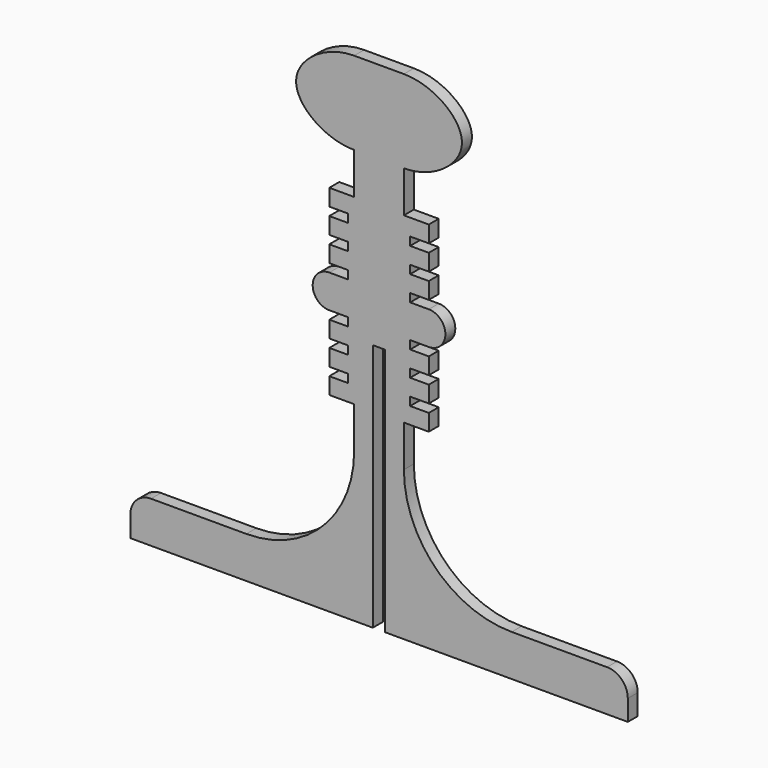
from build123d import *

# Parameters (mm, degrees)
F1_DEPTH = 3


# Not quite as in the source:
# - a feature names something its author has since deleted; it is built from what else it names


with BuildPart() as f1:
    # F0 (on Front) → F1 (new body)
    with BuildSketch(Plane.XZ):
        with BuildLine():
            Line((-1.5, 100), (-1.5, 120))
            Line((-1.5, 120), (-6, 120))
            add(Edge.make_bspline(
                [(-6, 120), (-13.1006129086, 120), (-20, 115.0061184168), (-20, 110)],
                knots=[0, 0, 0, 0, 0.5, 0.5, 0.5, 0.5], degree=3))
            add(Edge.make_bspline(
                [(-20, 110), (-20, 104.9938815832), (-13.1006129086, 99.9755263329), (-6, 100)],
                knots=[0.5, 0.5, 0.5, 0.5, 1, 1, 1, 1], degree=3))
            Line((-6, 100), (-1.5, 100))
        make_face()
        Polygon((-12, 68), (-6, 68), (-6, 90), (-12, 90), (-12, 86), (-7.5, 86), (-7.5, 84), (-12, 84), (-12, 80), (-7.5, 80), (-7.5, 78), (-12, 78), (-12, 74), (-7.5, 74), (-7.5, 72), (-12, 72), align=None)
        Polygon((-12, 46), (-6, 46), (-6, 68), (-12, 68), (-12, 64), (-7.5, 64), (-7.5, 62), (-12, 62), (-12, 58), (-7.5, 58), (-7.5, 56), (-12, 56), (-12, 52), (-7.5, 52), (-7.5, 50), (-12, 50), align=None)
        with BuildLine():
            Line((-12, 64), (-12, 68))
            Line((-12, 68), (-12, 72))
            ThreePointArc((-12, 72), (-16, 68), (-12, 64))
        make_face()
        with BuildLine():
            Line((12, 68), (12, 64))
            ThreePointArc((12, 64), (16, 68), (12, 72))
            Line((12, 72), (12, 68))
        make_face()
        Polygon((6, 90), (6, 46), (12, 46), (12, 50), (7.5, 50), (7.5, 52), (12, 52), (12, 56), (7.5, 56), (7.5, 58), (12, 58), (12, 62), (7.5, 62), (7.5, 64), (12, 64), (12, 68), (12, 72), (7.5, 72), (7.5, 74), (12, 74), (12, 78), (7.5, 78), (7.5, 80), (12, 80), (12, 84), (7.5, 84), (7.5, 86), (12, 86), (12, 90), align=None)
        with BuildLine():
            Line((1.5, 0), (60, 0))
            Line((60, 0), (60, 5))
            ThreePointArc((60, 5), (58.5355339059, 8.5355339059), (55, 10))
            Line((55, 10), (32, 10))
            ThreePointArc((32, 10), (13.6152236891, 17.6152236891), (6, 36))
            Line((6, 36), (6, 46))
            Line((6, 46), (6, 90))
            Line((6, 90), (6, 100))
            add(Edge.make_bspline(
                [(6, 120), (13.1006129086, 120), (26.8993870914, 110.0122368336), (13.1006129086, 99.9755263329), (6, 100)],
                knots=[0, 0, 0, 0, 0.5, 1, 1, 1, 1], degree=3))
            Line((6, 120), (1.5, 120))
            Line((1.5, 120), (-1.5, 120))
            Line((-1.5, 120), (-1.5, 100))
            Line((-1.5, 100), (-6, 100))
            Line((-6, 100), (-6, 90))
            Line((-6, 90), (-6, 68))
            Line((-6, 68), (-6, 46))
            Line((-6, 46), (-6, 36))
            ThreePointArc((-6, 36), (-13.6152236891, 17.6152236891), (-32, 10))
            Line((-32, 10), (-55, 10))
            ThreePointArc((-55, 10), (-58.5355339059, 8.5355339059), (-60, 5))
            Line((-60, 5), (-60, 0))
            Line((-60, 0), (-1.5, 0))
            Line((-1.5, 0), (-1.5, 60))
            Line((-1.5, 60), (1.5, 60))
            Line((1.5, 60), (1.5, 0))
        make_face()
    extrude(amount=F1_DEPTH)


solid = f1.part
